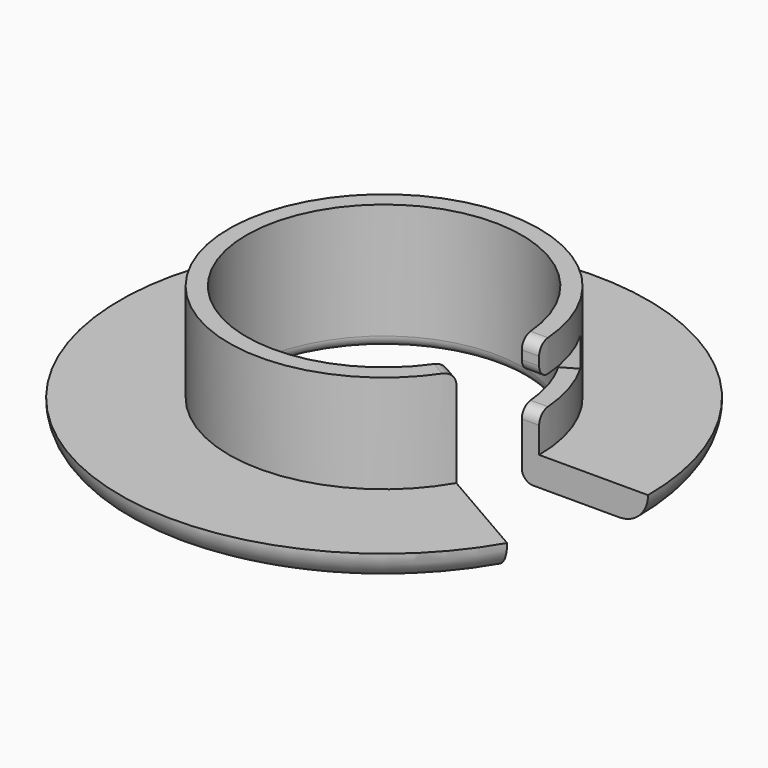
from build123d import *

# Parameters (mm, degrees)
F3_DEPTH      = 17.001
F3_DEPTH_BACK = 25
F6_DEPTH      = 2.5
F7_R          = 2
F8_DEPTH      = 1.8


with BuildPart() as f1:
    # F0 (on Front) → F1 (revolve)
    with BuildSketch(Plane.XZ):
        with BuildLine():
            Line((-23.8, 17), (-26.8, 17))
            Line((-26.8, 17), (-26.8, 0))
            Line((-26.8, 0), (-45.6279513852, 0))
            ThreePointArc((-45.6279513852, 0), (-44.1634852911, -3.5355339059), (-40.6279513852, -5))
            Line((-40.6279513852, -5), (-25.8, -5))
            ThreePointArc((-25.8, -5), (-24.3857864376, -4.4142135624), (-23.8, -3))
            Line((-23.8, -3), (-23.8, 17))
        make_face()
    revolve(axis=Axis((0, 0, 7.2955568321), (0, 0, 1)))

    # F2 (on Top) → F3 (cut, two sides)
    with BuildSketch(Plane.XY) as f3_sk:
        Polygon((53.3640757203, 0), (0, 0), (46.3265438035, -26.7466425355), align=None)
    extrude(amount=F3_DEPTH, mode=Mode.SUBTRACT)
    extrude(f3_sk.sketch, amount=-F3_DEPTH_BACK, mode=Mode.SUBTRACT)

    # F5 (on offset) → F6 (cut, symmetric)
    with BuildSketch(Plane.XY.offset(9)):
        Polygon((26.6670817875, 15.3962468485), (0, 0), (30.5216945708, 0), align=None)
    extrude(amount=F6_DEPTH, both=True, mode=Mode.SUBTRACT)

    # F7
    f7_edges = [f1.edges().sort_by_distance(p)[0] for p in [
        (21.910443, -12.65, 17),
        (25.3, 0, 17),
        (25.3, 0, 11.5),
        (25.3, 0, 6.5),
    ]]
    fillet(f7_edges, radius=F7_R)

    # F5 (on offset) → F8 (join, symmetric)
    with BuildSketch(Plane.XY.offset(9)):
        with BuildLine():
            Line((-21.9827251313, 12.2826441446), (-26.0146328451, 14.535435251))
            ThreePointArc((-26.0146328451, 14.535435251), (-27.6893290703, 11.0154916202), (-28.8902531983, 7.3070698737))
            Line((-28.8902531983, 7.3070698737), (-23.0896898866, 5.8399618793))
            Line((-23.0896898866, 5.8399618793), (-21.9827251313, 12.2826441446))
        make_face()
    extrude(amount=F8_DEPTH, both=True)


solid = f1.part
